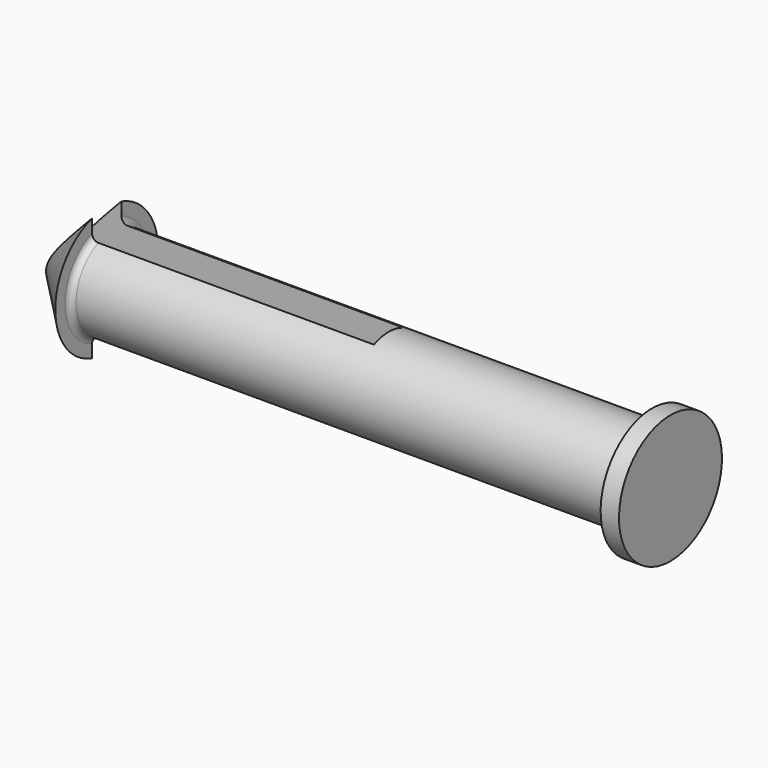
from build123d import *
from build123d import SkipClean  # not in build123d's __all__

# Parameters (mm, degrees)
F1_ANGLE_BACK = 90
F1_ANGLE      = 180
F2_ANGLE_BACK = 90
F2_ANGLE      = 180
F3_DEPTH      = 5.5
F4_R          = 0.5


with BuildPart() as f1:
    # F0 (on Top) → F1 (revolve)
    with BuildSketch(Plane.XY, mode=Mode.PRIVATE) as f1_sk:
        Polygon((23, 0), (0, 0), (0, -1.5), (0, -3.75), (21.5, -3.75), (21.5, -5.25), (23, -5.25), (23, -3.75), (23, -1.5), align=None)
        Polygon((0, -3.75), (0, -1.5), (-11.5, -1.5), (-23, -1.5), (-26.75, -1.5), (-23, -5.25), (-23, -3.75), align=None)
    revolve(f1_sk.sketch.rotate(Axis((11.5, 0, 0), (1, 0, 0)), -F1_ANGLE_BACK), axis=Axis((11.5, 0, 0), (1, 0, 0)), revolution_arc=F1_ANGLE)

    # F0 (on Top) → F2 (revolve)
    with BuildSketch(Plane.XY, mode=Mode.PRIVATE) as f2_sk:
        Polygon((21.5, 5.25), (21.5, 3.75), (11.5, 3.75), (0, 3.75), (0, 1.5), (0, 0), (23, 0), (23, 1.5), (23, 3.75), (23, 5.25), align=None)
        Polygon((0, 1.5), (0, 3.75), (-23, 3.75), (-23, 5.25), (-26.75, 1.5), (-23, 1.5), (-11.5, 1.5), align=None)
    revolve(f2_sk.sketch.rotate(Axis((11.5, 0, 0), (1, 0, 0)), -F2_ANGLE_BACK), axis=Axis((11.5, 0, 0), (1, 0, 0)), revolution_arc=F2_ANGLE)

    # F0 (on Top) → F3 (cut, symmetric)
    with BuildSketch(Plane.XY):
        Polygon((0, 0), (0, 1.5), (-11.5, 1.5), (-23, 1.5), (-26.75, 1.5), (-26.75, -1.5), (-23, -1.5), (-11.5, -1.5), (0, -1.5), align=None)
    with SkipClean():  # cleaning this boolean's faces spoils the solid; the shape is the same uncleaned
        extrude(amount=F3_DEPTH, both=True, mode=Mode.SUBTRACT)

    # F4
    f4_edges = [f1.edges().sort_by_distance(p)[0] for p in [
        (-23, 3.75, 0),
        (-23, -3.75, 0),
    ]]
    fillet(f4_edges, radius=F4_R)


solid = f1.part
